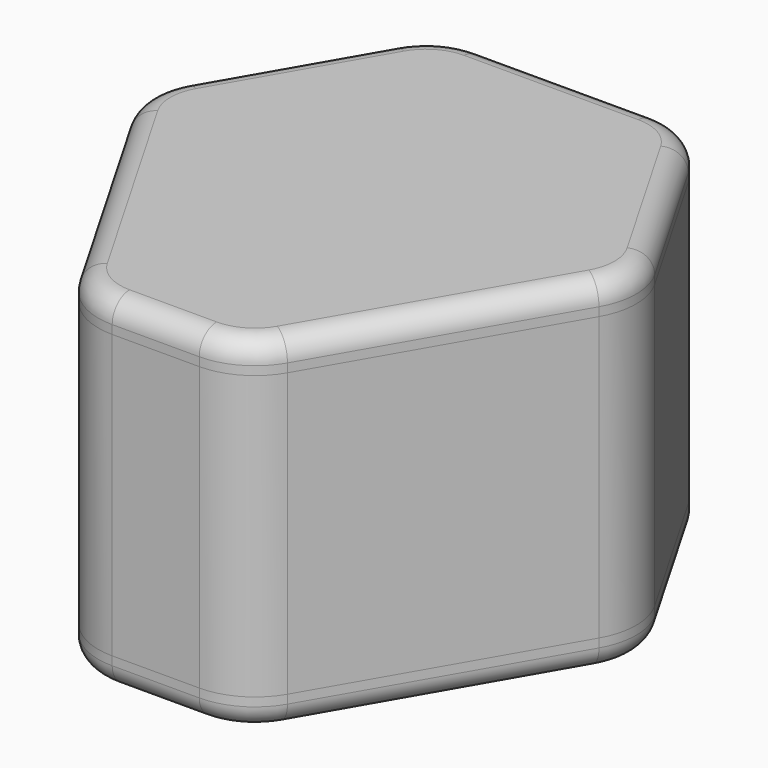
from build123d import *

# Parameters (mm, degrees)
F0_R     = 9
F1_DEPTH = 65
F2_R     = 2
F4_DEPTH = 65
F6_DEPTH = 5
F8_DEPTH = 2
F9_R     = 4.99999


# Not quite as in the source:
# - a fillet or chamfer is up to 0.001 mm smaller than in the source, because OpenCascade refuses the exact size


with BuildPart() as f1:
    # F0 (on Top) → F1 (new body)
    with BuildSketch(Plane.XY):
        Circle(F0_R)
    extrude(amount=F1_DEPTH)

    # F2
    f2_edges = [f1.edges().sort_by_distance(p)[0] for p in [
        (-9, 0, 65),
        (-9, 0, 0),
    ]]
    fillet(f2_edges, radius=F2_R)


with BuildPart() as f4:
    # F3 (on Top) → F4 (new body)
    with BuildSketch(Plane.XY):
        with BuildLine():
            Line((60, 50.6410161514), (20, 50.6410161514))
            ThreePointArc((20, 50.6410161514), (12, 48.4974226119), (6.1435935394, 42.6410161514))
            Line((6.1435935394, 42.6410161514), (-13.8564064606, 8))
            ThreePointArc((-13.8564064606, 8), (-16, 0), (-13.8564064606, -8))
            Line((-13.8564064606, -8), (16.1435935394, -59.9615242271))
            ThreePointArc((16.1435935394, -59.9615242271), (22, -65.8179306876), (30, -67.9615242271))
            Line((30, -67.9615242271), (50, -67.9615242271))
            ThreePointArc((50, -67.9615242271), (58, -65.8179306876), (63.8564064606, -59.9615242271))
            Line((63.8564064606, -59.9615242271), (93.8564064606, -8))
            ThreePointArc((93.8564064606, -8), (96, 0), (93.8564064606, 8))
            Line((93.8564064606, 8), (73.8564064606, 42.6410161514))
            ThreePointArc((73.8564064606, 42.6410161514), (68, 48.4974226119), (60, 50.6410161514))
        make_face()
        with BuildLine():
            ThreePointArc((7.875644347, 41.6410161514), (13, 46.7653718044), (20, 48.6410161514))
            Line((20, 48.6410161514), (60, 48.6410161514))
            ThreePointArc((60, 48.6410161514), (67, 46.7653718044), (72.124355653, 41.6410161514))
            Line((72.124355653, 41.6410161514), (92.124355653, 7))
            ThreePointArc((92.124355653, 7), (94, 0), (92.124355653, -7))
            Line((92.124355653, -7), (62.124355653, -58.9615242271))
            ThreePointArc((62.124355653, -58.9615242271), (57, -64.08587988), (50, -65.9615242271))
            Line((50, -65.9615242271), (30, -65.9615242271))
            ThreePointArc((30, -65.9615242271), (23, -64.08587988), (17.875644347, -58.9615242271))
            Line((17.875644347, -58.9615242271), (-12.124355653, -7))
            ThreePointArc((-12.124355653, -7), (-14, 0), (-12.124355653, 7))
            Line((-12.124355653, 7), (7.875644347, 41.6410161514))
        make_face(mode=Mode.SUBTRACT)
    extrude(amount=F4_DEPTH)


with BuildPart() as f6:
    # F5 (on face) → F6 (new body)
    with BuildSketch(Plane.XY.offset(65)):
        with BuildLine():
            Line((30, -67.9615242271), (50, -67.9615242271))
            ThreePointArc((50, -67.9615242271), (58, -65.8179306876), (63.8564064606, -59.9615242271))
            Line((63.8564064606, -59.9615242271), (93.8564064606, -8))
            ThreePointArc((93.8564064606, -8), (96, 0), (93.8564064606, 8))
            Line((93.8564064606, 8), (73.8564064606, 42.6410161514))
            ThreePointArc((73.8564064606, 42.6410161514), (68, 48.4974226119), (60, 50.6410161514))
            Line((60, 50.6410161514), (20, 50.6410161514))
            ThreePointArc((20, 50.6410161514), (12, 48.4974226119), (6.1435935394, 42.6410161514))
            Line((6.1435935394, 42.6410161514), (-13.8564064606, 8))
            ThreePointArc((-13.8564064606, 8), (-16, 0), (-13.8564064606, -8))
            Line((-13.8564064606, -8), (16.1435935394, -59.9615242271))
            ThreePointArc((16.1435935394, -59.9615242271), (22, -65.8179306876), (30, -67.9615242271))
        make_face()
        with BuildLine():
            Line((-12.124355653, 7), (7.875644347, 41.6410161514))
            ThreePointArc((7.875644347, 41.6410161514), (13, 46.7653718044), (20, 48.6410161514))
            Line((20, 48.6410161514), (60, 48.6410161514))
            ThreePointArc((60, 48.6410161514), (67, 46.7653718044), (72.124355653, 41.6410161514))
            Line((72.124355653, 41.6410161514), (92.124355653, 7))
            ThreePointArc((92.124355653, 7), (94, 0), (92.124355653, -7))
            Line((92.124355653, -7), (62.124355653, -58.9615242271))
            ThreePointArc((62.124355653, -58.9615242271), (57, -64.08587988), (50, -65.9615242271))
            Line((50, -65.9615242271), (30, -65.9615242271))
            ThreePointArc((30, -65.9615242271), (23, -64.08587988), (17.875644347, -58.9615242271))
            Line((17.875644347, -58.9615242271), (-12.124355653, -7))
            ThreePointArc((-12.124355653, -7), (-14, 0), (-12.124355653, 7))
        make_face(mode=Mode.SUBTRACT)
    extrude(amount=F6_DEPTH)

    # F7 (on face) → F8 (join)
    with BuildSketch(Plane.XY.offset(70)):
        with BuildLine():
            ThreePointArc((16.1435935394, -59.9615242271), (22, -65.8179306876), (30, -67.9615242271))
            Line((30, -67.9615242271), (50, -67.9615242271))
            ThreePointArc((50, -67.9615242271), (58, -65.8179306876), (63.8564064606, -59.9615242271))
            Line((63.8564064606, -59.9615242271), (93.8564064606, -8))
            ThreePointArc((93.8564064606, -8), (96, 0), (93.8564064606, 8))
            Line((93.8564064606, 8), (73.8564064606, 42.6410161514))
            ThreePointArc((73.8564064606, 42.6410161514), (68, 48.4974226119), (60, 50.6410161514))
            Line((60, 50.6410161514), (20, 50.6410161514))
            ThreePointArc((20, 50.6410161514), (12, 48.4974226119), (6.1435935394, 42.6410161514))
            Line((6.1435935394, 42.6410161514), (-13.8564064606, 8))
            ThreePointArc((-13.8564064606, 8), (-16, 0), (-13.8564064606, -8))
            Line((-13.8564064606, -8), (16.1435935394, -59.9615242271))
        make_face()
        with BuildLine():
            ThreePointArc((30, -65.9615242271), (23, -64.08587988), (17.875644347, -58.9615242271))
            Line((17.875644347, -58.9615242271), (-12.124355653, -7))
            ThreePointArc((-12.124355653, -7), (-14, 0), (-12.124355653, 7))
            Line((-12.124355653, 7), (7.875644347, 41.6410161514))
            ThreePointArc((7.875644347, 41.6410161514), (13, 46.7653718044), (20, 48.6410161514))
            Line((20, 48.6410161514), (60, 48.6410161514))
            ThreePointArc((60, 48.6410161514), (67, 46.7653718044), (72.124355653, 41.6410161514))
            Line((72.124355653, 41.6410161514), (92.124355653, 7))
            ThreePointArc((92.124355653, 7), (94, 0), (92.124355653, -7))
            Line((92.124355653, -7), (62.124355653, -58.9615242271))
            ThreePointArc((62.124355653, -58.9615242271), (57, -64.08587988), (50, -65.9615242271))
            Line((50, -65.9615242271), (30, -65.9615242271))
        make_face(mode=Mode.SUBTRACT)
        with BuildLine():
            Line((-12.124355653, -7), (17.875644347, -58.9615242271))
            ThreePointArc((17.875644347, -58.9615242271), (23, -64.08587988), (30, -65.9615242271))
            Line((30, -65.9615242271), (50, -65.9615242271))
            ThreePointArc((50, -65.9615242271), (57, -64.08587988), (62.124355653, -58.9615242271))
            Line((62.124355653, -58.9615242271), (92.124355653, -7))
            ThreePointArc((92.124355653, -7), (94, 0), (92.124355653, 7))
            Line((92.124355653, 7), (72.124355653, 41.6410161514))
            ThreePointArc((72.124355653, 41.6410161514), (67, 46.7653718044), (60, 48.6410161514))
            Line((60, 48.6410161514), (20, 48.6410161514))
            ThreePointArc((20, 48.6410161514), (13, 46.7653718044), (7.875644347, 41.6410161514))
            Line((7.875644347, 41.6410161514), (-12.124355653, 7))
            ThreePointArc((-12.124355653, 7), (-14, 0), (-12.124355653, -7))
        make_face()
    extrude(amount=F8_DEPTH)

    # F9 (radius 5 in the source; OpenCascade refuses exactly that, so slightly less here)
    f9_edges = [f6.edges().sort_by_distance(p)[0] for p in [
        (-3.856406, 25.320508, 72),
        (67, 46.765372, 70),
    ]]
    fillet(f9_edges, radius=F9_R)


with BuildPart() as f11_1:
    # F11: instance of F6
    add(f6.part.mirror(Plane.XY.offset(32.5)))


solid = Compound([f1.part, f4.part, f6.part, f11_1.part])
